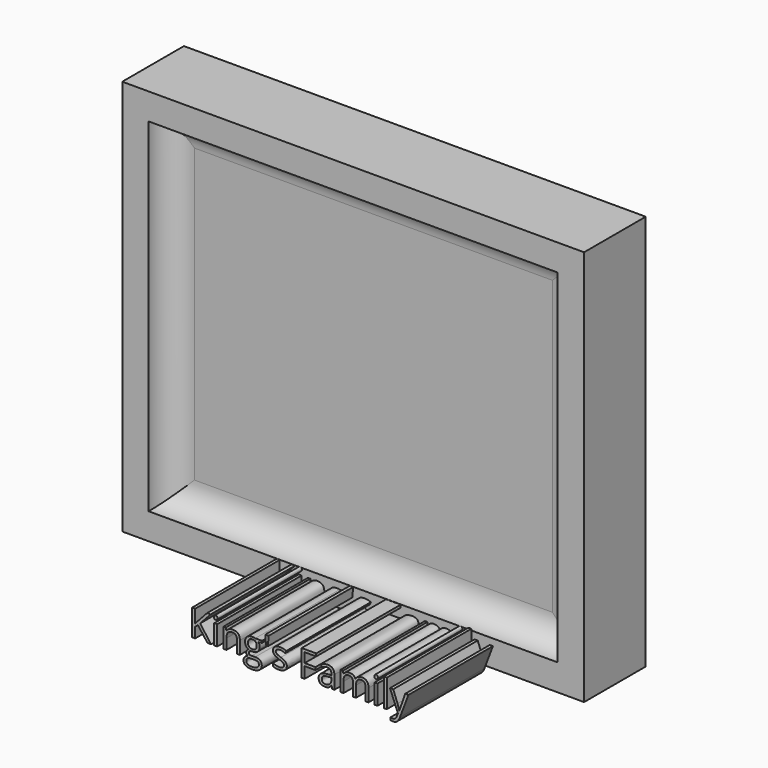
from build123d import *

# Parameters (mm, degrees)
F1_DEPTH     = 12.446
F2_W         = 111.093018204
F2_H         = 95.2637046576
F2_W_2       = 98.3930192888
F2_H_2       = 82.5637057424
F3_DEPTH     = 6.096
F4_T4_DEPTH  = 98.3930192888
F4_T9_DEPTH  = 82.5637057424
F4_T14_DEPTH = 98.3930192888
F4_T19_DEPTH = 82.5637057424
F5_TEXT_SIZE = 8.8194436911
F6_DEPTH     = 25.4


# Not quite as in the source:
# - a fillet or chamfer that OpenCascade refuses, or shapes differently, is made with other operations: its cross-section is extruded or revolved along the edge and cut away or added
# - Text() gives the source's letters only with a copy of the font that has no kerning and outlines rounded to 1/6400 em; it was checked with that copy


with BuildPart() as f1:
    # F0 (on Front) → F1 (new body)
    with BuildSketch(Plane.XZ):
        Polygon((-57.705052197, 55.1148019731), (-57.705052197, 0), (-57.705052197, -40.1489026845), (53.387966007, -40.1489026845), (53.387966007, 55.1148019731), align=None)
    extrude(amount=F1_DEPTH)

    # F2 (on face) → F3 (join)
    with BuildSketch(Plane.XZ.offset(12.446)):
        with Locations((-2.158543095, 7.4829496443)):
            Rectangle(F2_W, F2_H)
        with Locations((-2.158543095, 7.4829496443)):
            Rectangle(F2_W_2, F2_H_2, mode=Mode.SUBTRACT)
    extrude(amount=F3_DEPTH)

    # F4: fillet of radius 6.1321024484 on 4 edges, made by hand


with BuildPart() as f4_tool2:
    # F4_s3 → F4_t4 (new body)
    with BuildSketch(Plane.YZ.offset(-51.3550527394)):
        with BuildLine():
            ThreePointArc((-12.446, 42.6327000671), (-14.2420512242, 46.9687512913), (-18.5781024484, 48.7648025155))
            Line((-18.5781024484, 48.7648025155), (-12.446, 48.7648025155))
            Line((-12.446, 48.7648025155), (-12.446, 42.6327000671))
        make_face()
    extrude(amount=F4_T4_DEPTH)

    split(bisect_by=Plane.XZ.offset(18.542), keep=Keep.BOTTOM)


with BuildPart() as f1_1:
    add(f1.part)

    # F4_t1: union F4_tool2
    add(f4_tool2.part)


with BuildPart() as f4_tool7:
    # F4_s8 → F4_t9 (new body)
    with BuildSketch(Plane.XY.offset(48.7648025155)):
        with BuildLine():
            ThreePointArc((40.905864101, -12.446), (45.2419153252, -14.2420512242), (47.0379665494, -18.5781024484))
            Line((47.0379665494, -18.5781024484), (47.0379665494, -12.446))
            Line((47.0379665494, -12.446), (40.905864101, -12.446))
        make_face()
    extrude(amount=-F4_T9_DEPTH)

    split(bisect_by=Plane.XZ.offset(18.542), keep=Keep.BOTTOM)


with BuildPart() as f1_2:
    add(f1_1.part)

    # F4_t6: union F4_tool7
    add(f4_tool7.part)


with BuildPart() as f4_tool12:
    # F4_s13 → F4_t14 (new body)
    with BuildSketch(Plane.YZ.offset(47.0379665494)):
        with BuildLine():
            ThreePointArc((-12.446, -27.6668007784), (-14.2420512242, -32.0028520026), (-18.5781024484, -33.7989032269))
            Line((-18.5781024484, -33.7989032269), (-12.446, -33.7989032269))
            Line((-12.446, -33.7989032269), (-12.446, -27.6668007784))
        make_face()
    extrude(amount=-F4_T14_DEPTH)

    split(bisect_by=Plane.XZ.offset(18.542), keep=Keep.BOTTOM)


with BuildPart() as f1_3:
    add(f1_2.part)

    # F4_t11: union F4_tool12
    add(f4_tool12.part)


with BuildPart() as f4_tool17:
    # F4_s18 → F4_t19 (new body)
    with BuildSketch(Plane.XY.offset(-33.7989032269)):
        with BuildLine():
            ThreePointArc((-51.3550527394, -18.5781024484), (-49.5590015152, -14.2420512242), (-45.222950291, -12.446))
            Line((-45.222950291, -12.446), (-51.3550527394, -12.446))
            Line((-51.3550527394, -12.446), (-51.3550527394, -18.5781024484))
        make_face()
    extrude(amount=F4_T19_DEPTH)

    split(bisect_by=Plane.XZ.offset(18.542), keep=Keep.BOTTOM)


with BuildPart() as f1_4:
    add(f1_3.part)

    # F4_t16: union F4_tool17
    add(f4_tool17.part)


with BuildPart() as f6:
    # F5 (on face) → F6 (new body)
    with BuildSketch(Plane.XZ.offset(18.542)):
        with Locations((-21.4415285736, -40.1489026845)):
            Text("King's Family", F5_TEXT_SIZE, font='Open Sans', text_align=(TextAlign.LEFT, TextAlign.BOTTOM))
    extrude(amount=F6_DEPTH)


solid = Compound([f1_4.part, f6.part])
